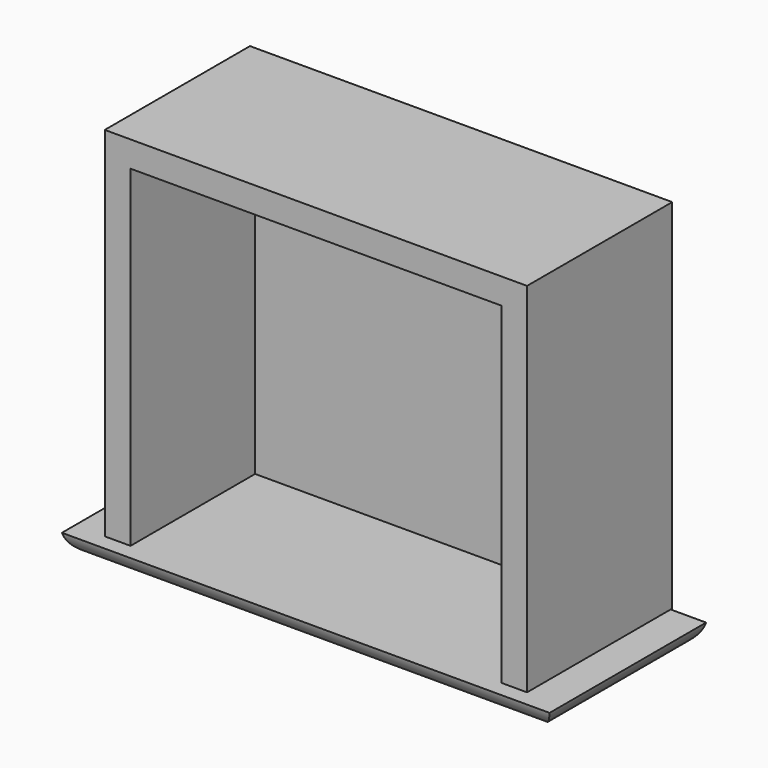
from build123d import *

# Parameters (mm, degrees)
F0_W        = 83.3283886313
F0_H        = 70.6079043448
F1_DEPTH    = 35.814
F2_T        = -5.08
F3_W        = 96.2229035795
F3_H        = 3.9905235171
F4_DEPTH    = 38.608
F5_T1_DEPTH = 121.0318943859
F5_T3_DEPTH = 63.4169908064


# Not quite as in the source:
# - a fillet or chamfer that OpenCascade refuses, or shapes differently, is made with other operations: its cross-section is extruded or revolved along the edge and cut away or added


with BuildPart() as f1:
    # F0 (on Front) → F1 (new body)
    with BuildSketch(Plane.XZ):
        with Locations((1.751370728, 0.5530659109)):
            Rectangle(F0_W, F0_H)
    extrude(amount=F1_DEPTH)

    # F2
    f2_openings = [f1.faces().sort_by_distance(p)[0] for p in [
        (1.751371, -35.814, 0.553066),
        (1.751371, -17.907, -34.750886),
    ]]
    offset(amount=F2_T, openings=f2_openings)


with BuildPart() as f4:
    # F3 (on Front) → F4 (new body)
    with BuildSketch(Plane.XZ):
        with Locations((1.980105415, -37.0091460645)):
            Rectangle(F3_W, F3_H)
    extrude(amount=F4_DEPTH)

    # F5: fillet of radius 5.08 on 4 edges, made by hand

    # F5_s2 → F5_t1 (cut)
    with BuildSketch(Plane.YZ.offset(-58.5358417779)):
        with BuildLine():
            ThreePointArc((-33.6462018387, -39.0044078231), (-36.8298993328, -37.8830023043), (-38.608, -35.013884306))
            Line((-38.608, -35.013884306), (-38.608, -39.0044078231))
            Line((-38.608, -39.0044078231), (-33.6462018387, -39.0044078231))
        make_face()
        with BuildLine():
            ThreePointArc((-4.9617981613, -39.0044078231), (-1.7781006672, -37.8830023043), (0, -35.013884306))
            Line((0, -35.013884306), (0, -39.0044078231))
            Line((0, -39.0044078231), (-4.9617981613, -39.0044078231))
        make_face()
    extrude(amount=F5_T1_DEPTH, mode=Mode.SUBTRACT)

    # F5_s4 → F5_t3 (cut)
    with BuildSketch(Plane.XZ.offset(-12.4044954032)):
        with BuildLine():
            ThreePointArc((45.1297590434, -39.0044078231), (48.3134565375, -37.8830023043), (50.0915572047, -35.013884306))
            Line((50.0915572047, -35.013884306), (50.0915572047, -39.0044078231))
            Line((50.0915572047, -39.0044078231), (45.1297590434, -39.0044078231))
        make_face()
        with BuildLine():
            ThreePointArc((-46.1313463748, -35.013884306), (-44.3532457075, -37.8830023043), (-41.1695482135, -39.0044078231))
            Line((-41.1695482135, -39.0044078231), (-46.1313463748, -39.0044078231))
            Line((-46.1313463748, -39.0044078231), (-46.1313463748, -35.013884306))
        make_face()
    extrude(amount=F5_T3_DEPTH, mode=Mode.SUBTRACT)


with BuildPart() as f7:
    # F6 (on Right) → F7 (revolve)
    with BuildSketch(Plane.YZ):
        with BuildLine():
            Line((-18.7280923128, -39.2518080771), (-19.8871381581, -39.2518080771))
            Line((-19.8871381581, -39.2518080771), (-19.8871381581, -45.8132699132))
            add(Edge.make_bspline(
                [(-19.8871381581, -45.8132699132), (-13.5188465938, -44.8499545455), (-19.8871381581, -40.5852496624), (-18.7280923128, -39.2518080771)],
                knots=[0, 0, 0, 0, 6.663045002, 6.663045002, 6.663045002, 6.663045002], degree=3))
        make_face()
    revolve(axis=Axis((0, -19.8871381581, -42.5325389951), (0, 0, -1)))


solid = Compound([f1.part, f4.part, f7.part])
